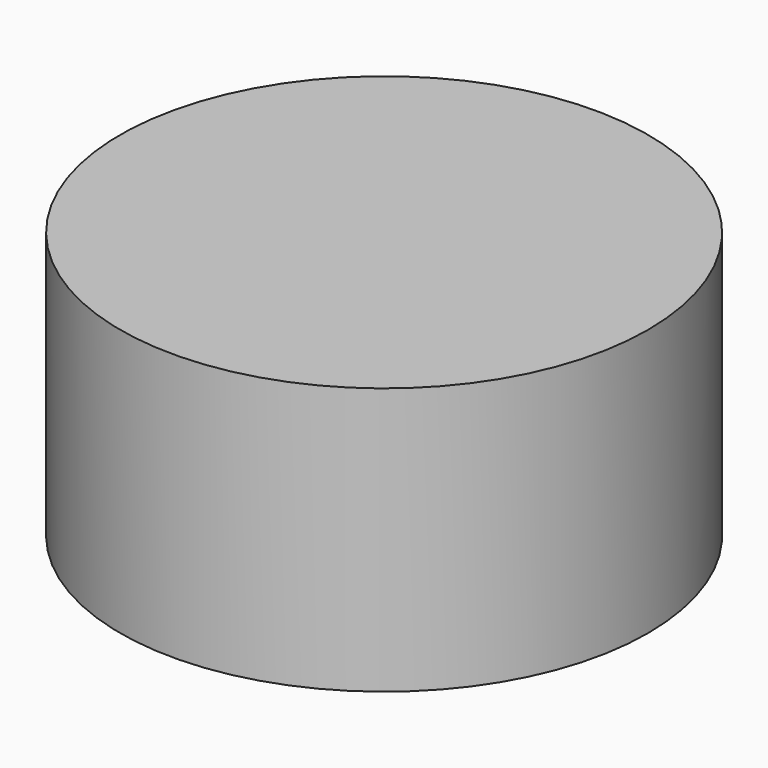
from build123d import *

# Parameters (mm, degrees)
F0_R     = 25.1094331867
F1_DEPTH = 25.4


# Not quite as in the source:
# - the program builds the solid bodies; features that only make, move or delete a surface that nothing else refers to are left out


with BuildPart() as f1:
    # F0 (on Top) → F1 (new body)
    with BuildSketch(Plane.XY):
        with Locations((3.0484944582, -1.9060224295)):
            Circle(F0_R)
    extrude(amount=F1_DEPTH)


solid = f1.part
